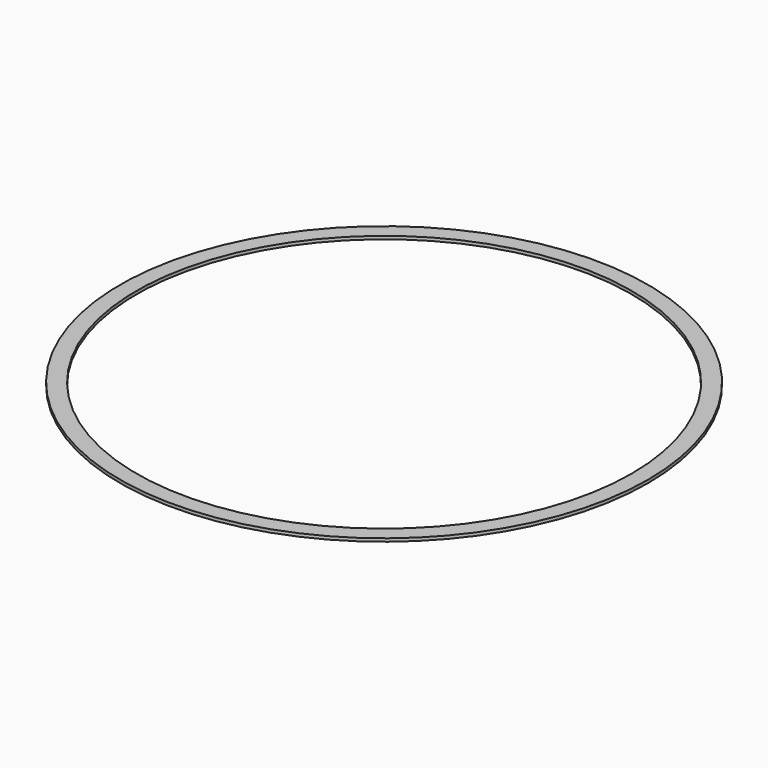
from build123d import *

# Parameters (mm, degrees)
F0_R     = 409.02509
F0_R_2   = 383.62509
F1_DEPTH = 4.7625


# Not quite as in the source:
# - a length typed as a fraction of an inch, garbled in the dataset ("3 / 203.2 mm" for 3/8 in), is restored


with BuildPart() as f1:
    # F0 (on Top) → F1 (new body)
    with BuildSketch(Plane.XY):
        Circle(F0_R)
        Circle(F0_R_2, mode=Mode.SUBTRACT)
    extrude(amount=F1_DEPTH)


solid = f1.part
